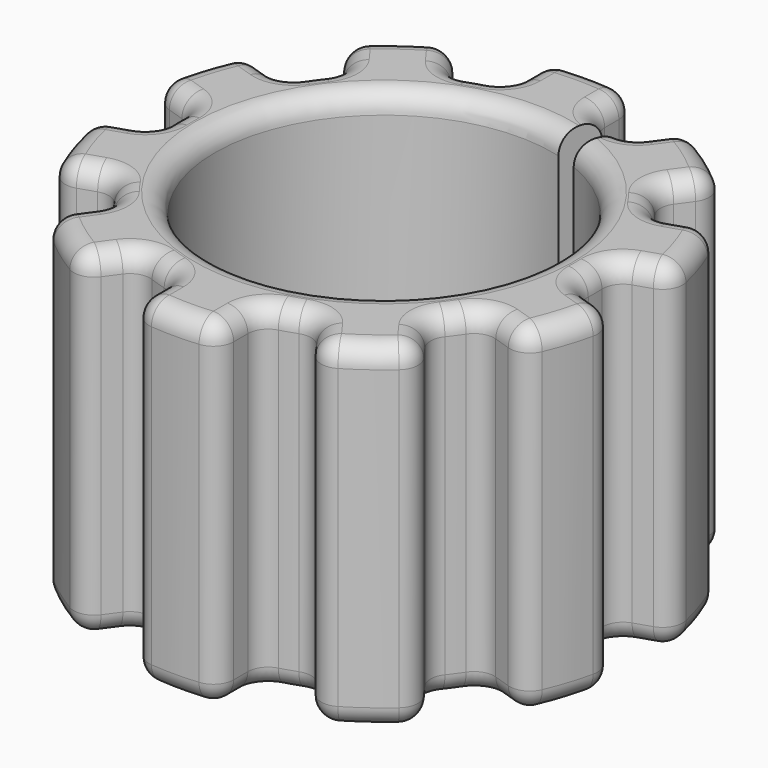
from build123d import *

# Parameters (mm, degrees)
F0_R            = 12.5
F0_R_2          = 10
F1_DEPTH        = 20
F3_DEPTH        = 20
F3_COPIES_COUNT = 10
F4_R            = 1.2
F6_R            = 1.2
F8_DEPTH        = 20.001


# Not quite as in the source:
# - a pattern or mirror of a feature is missing from the dataset's text; its kind, count and spacing are read off the source's solid


with BuildPart() as f1:
    # F0 (on Top) → F1 (new body)
    with BuildSketch(Plane.XY):
        Circle(F0_R)
        Circle(F0_R_2, mode=Mode.SUBTRACT)
    extrude(amount=F1_DEPTH)

    # F2 (on face) → F3 (join, through all)
    with BuildSketch(Plane.XY.offset(20)):
        with BuildLine():
            Line((2.5, 12.2474487139), (2.5, 15.2970585408))
            ThreePointArc((2.5, 15.2970585408), (0, 15.5), (-2.5, 15.2970585408))
            Line((-2.5, 15.2970585408), (-2.5, 12.2474487139))
            ThreePointArc((-2.5, 12.2474487139), (0, 12.5), (2.5, 12.2474487139))
        make_face()
    f3 = extrude(amount=-F3_DEPTH)

    # F3_copies: F3 ×10 about axis
    f3_copies_axis = Axis((0, 0, 0), (0, 0, 1))
    for i in range(1, F3_COPIES_COUNT):
        add(f3.rotate(f3_copies_axis, i * 360 / F3_COPIES_COUNT))

    # F4
    f4_edges = [f1.edges().sort_by_distance(p)[0] for p in [
        (-2.5, 12.247449, 10),
        (-2.5, 15.297059, 10),
        (2.5, 15.297059, 10),
        (2.5, 12.247449, 10),
    ]]
    fillet(f4_edges, radius=F4_R)

    # F6
    f6_edges = [f1.edges().sort_by_distance(p)[0] for p in [
        (-10, 0, 20),
        (-4.288744, 11.741238, 0),
        (-5.176327, 11.377857, 10),
        (-4.288744, 11.741238, 20),
        (2.5, 13.715846, 0),
        (2.74373, 12.465959, 0),
        (2.186259, 15.049826, 0),
        (0, 15.5, 0),
        (6.072585, 12.61145, 0),
        (-2.186259, 15.049826, 0),
        (9.110671, 12.539763, 0),
        (-2.5, 13.715846, 0),
        (10.11767, 9.672524, 0),
        (-2.74373, 12.465959, 0),
        (10.112712, 7.347316, 0),
        (12.325649, 6.633502, 0),
        (-6.072585, 12.61145, 0),
        (14.741376, 4.789763, 0),
        (-9.110671, 12.539763, 0),
        (13.870734, 1.878219, 0),
        (-10.11767, 9.672524, 0),
        (12.5, 0, 0),
        (-10.112712, 7.347316, 0),
        (13.870734, -1.878219, 0),
        (-12.325649, 6.633502, 0),
        (14.741376, -4.789763, 0),
        (-14.741376, 4.789763, 0),
        (12.325649, -6.633502, 0),
        (-13.870734, 1.878219, 0),
        (10.112712, -7.347316, 0),
        (-12.5, 0, 0),
        (10.11767, -9.672524, 0),
        (-13.870734, -1.878219, 0),
        (9.110671, -12.539763, 0),
        (-14.741376, -4.789763, 0),
        (6.072585, -12.61145, 0),
        (-12.325649, -6.633502, 0),
        (3.862712, -11.888206, 0),
        (-10.112712, -7.347316, 0),
        (2.5, -13.772254, 0),
        (-10.11767, -9.672524, 0),
        (0, -15.5, 0),
        (-9.110671, -12.539763, 0),
        (-2.5, -13.772254, 0),
        (-6.072585, -12.61145, 0),
        (-3.862712, -11.888206, 0),
        (-10, 0, 0),
        (-2.74373, 12.465959, 20),
        (-6.968843, 13.845043, 10),
        (-6.072585, 12.61145, 20),
        (2.74373, 12.465959, 20),
        (6.072585, 12.61145, 20),
        (2.5, 13.715846, 20),
        (9.110671, 12.539763, 20),
        (2.186259, 15.049826, 20),
        (10.11767, 9.672524, 20),
        (0, 15.5, 20),
        (10.112712, 7.347316, 20),
        (-2.186259, 15.049826, 20),
        (12.325649, 6.633502, 20),
        (-2.5, 13.715846, 20),
        (14.741376, 4.789763, 20),
        (13.870734, 1.878219, 20),
        (12.5, 0, 20),
        (13.870734, -1.878219, 20),
        (-9.110671, 12.539763, 20),
        (14.741376, -4.789763, 20),
        (-10.11767, 9.672524, 20),
        (12.325649, -6.633502, 20),
        (-10.112712, 7.347316, 20),
        (10.112712, -7.347316, 20),
        (-12.325649, 6.633502, 20),
        (10.11767, -9.672524, 20),
        (-14.741376, 4.789763, 20),
        (9.110671, -12.539763, 20),
        (-13.870734, 1.878219, 20),
        (6.072585, -12.61145, 20),
        (-12.5, 0, 20),
        (3.862712, -11.888206, 20),
        (-13.870734, -1.878219, 20),
        (2.5, -13.772254, 20),
        (-14.741376, -4.789763, 20),
        (0, -15.5, 20),
        (-12.325649, -6.633502, 20),
        (-2.5, -13.772254, 20),
        (-10.112712, -7.347316, 20),
        (-3.862712, -11.888206, 20),
        (-10.11767, -9.672524, 20),
        (-6.072585, -12.61145, 20),
        (-9.110671, -12.539763, 20),
        (5.176327, 11.377857, 10),
        (6.968843, 13.845043, 10),
        (11.013928, 10.906117, 10),
        (9.221412, 8.438931, 10),
        (10.875473, 6.162311, 10),
        (13.775825, 7.104692, 10),
        (15.32091, 2.34941, 10),
        (-11.013928, 10.906117, 10),
        (12.420558, 1.407028, 10),
        (-9.221412, 8.438931, 10),
        (12.420558, -1.407028, 10),
        (-10.875473, 6.162311, 10),
        (15.32091, -2.34941, 10),
        (-13.775825, 7.104692, 10),
        (13.775825, -7.104692, 10),
        (-15.32091, 2.34941, 10),
        (10.875473, -6.162311, 10),
        (-12.420558, 1.407028, 10),
        (9.221412, -8.438931, 10),
        (-12.420558, -1.407028, 10),
        (11.013928, -10.906117, 10),
        (-15.32091, -2.34941, 10),
        (6.968843, -13.845043, 10),
        (-13.775825, -7.104692, 10),
        (5.176327, -11.377857, 10),
        (-10.875473, -6.162311, 10),
        (2.5, -12.247449, 10),
        (-9.221412, -8.438931, 10),
        (2.5, -15.297059, 10),
        (-11.013928, -10.906117, 10),
        (-2.5, -15.297059, 10),
        (-6.968843, -13.845043, 10),
        (-2.5, -12.247449, 10),
        (-5.176327, -11.377857, 10),
    ]]
    fillet(f6_edges, radius=F6_R)

    # F7 (on face) → F8 (cut, through all)
    with BuildSketch(Plane.XY.offset(20)):
        Polygon((8.0755222589, 30.0816278905), (0, 0), (11.4385781141, 27.5784555979), align=None)
    extrude(amount=-F8_DEPTH, mode=Mode.SUBTRACT)


solid = f1.part
